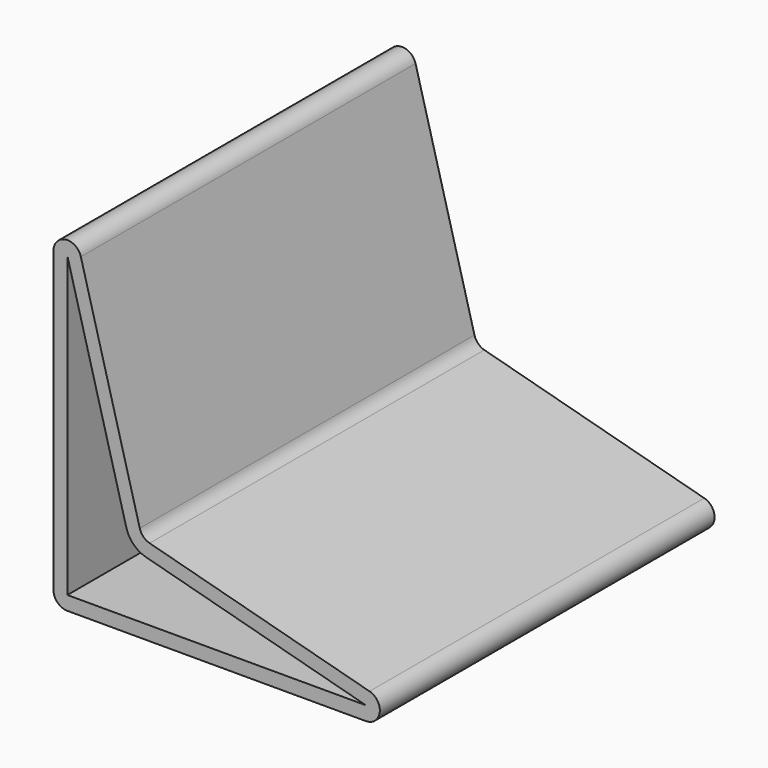
from build123d import *

# Parameters (mm, degrees)
F1_DEPTH = 76.2
F2_R     = 2.54
F3_T     = 2.54


# Not quite as in the source:
# - a shell that OpenCascade refuses in one call is made with other operations: the cavity is built on its own and cut out


with BuildPart() as f1:
    # F0 (on Front) → F1 (new body)
    with BuildSketch(Plane.XZ):
        Polygon((16.1029547439, 16.1029547439), (0, 76.2), (0, 0), (76.2, 0), align=None)
    extrude(amount=F1_DEPTH)

    # F2
    f2_edges = [f1.edges().sort_by_distance(p)[0] for p in [
        (0, -38.1, 76.2),
        (76.2, -38.1, 0),
        (16.102955, -38.1, 16.102955),
        (0, -38.1, 0),
    ]]
    fillet(f2_edges, radius=F2_R)

    # F3: shell of thickness 2.54, made by hand


with BuildPart() as f3_core1:
    # F3_t2: copy of F1
    add(f1.part)

    # the walls: a layer under each face that stays
    f3_faces = [f3_core1.faces().sort_by_distance(p)[0] for p in [
        (10.3584280297, -38.1, 37.5418203066),
        (9.9077974256, 0, 9.9077974256),
        (16.3808048352, -38.1, 16.3808048352),
        (37.5418203066, -38.1, 10.3584280297),
        (0, -38.1, 29.7233922768),
        (29.7233922768, -38.1, 0),
    ]]
    thicken(f3_faces, amount=-F3_T, mode=Mode.SUBTRACT)


with BuildPart() as f1_1:
    add(f1.part)

    # what is left inside the walls is the cavity
    f3_cavity = [f3_core1.part.solids().sort_by_distance(p)[0] for p in [
        (29.723392, -51.646667, 2.5654),
    ]]
    add(f3_cavity, mode=Mode.SUBTRACT)


solid = f1_1.part
